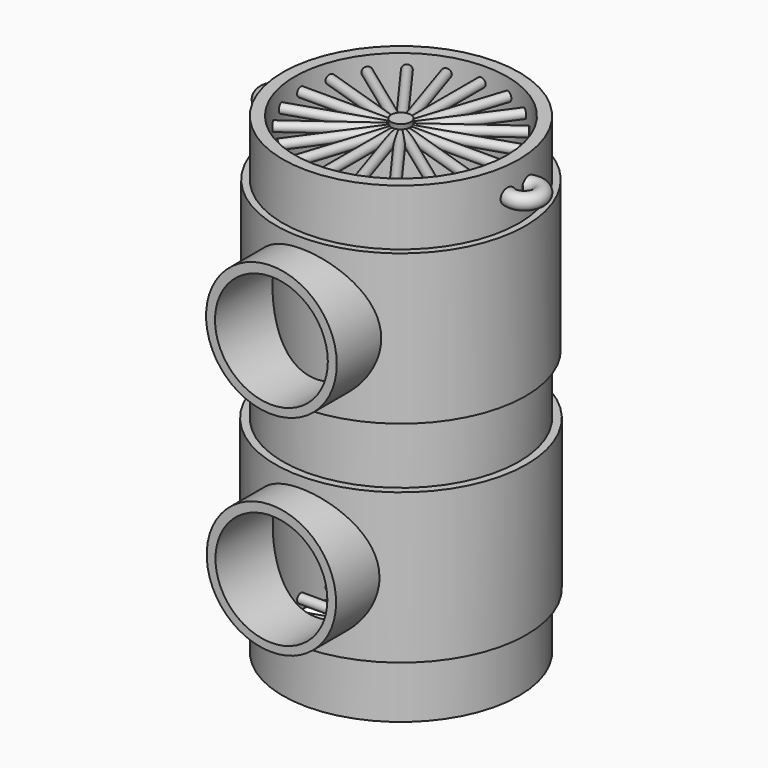
from build123d import *

# Parameters (mm, degrees)
F0_R      = 50
F1_DEPTH  = 100
F3_R      = 52.8567607849
F4_DEPTH  = 63.5
F6_R      = 53.2150165933
F7_DEPTH  = 63.5
F9_R      = 27.6777102691
F9_R_2    = 27.4003566056
F11_R     = 44.9963052647
F12_DEPTH = 104.14
F13_R     = 23.8902101051
F13_R_2   = 23.6973666463
F14_DEPTH = 30.4506270542
F16_R     = 4.1676041999
F17_DEPTH = 10
F18_R     = 1.9662297222
F19_DEPTH = 42.418
F20_COUNT = 20
F22_R     = 4.1676041999
F23_DEPTH = 10
F24_R     = 1.9662297222
F25_DEPTH = 42.418
F26_COUNT = 20
F27_R     = 3.2683339777
F31_R     = 3.2683339777


with BuildPart() as f1:
    # F0 (on Top) → F1 (new body, symmetric)
    with BuildSketch(Plane.XY):
        Circle(F0_R)
    extrude(amount=F1_DEPTH, both=True)

    # F3 (on offset) → F4 (join)
    with BuildSketch(Plane.XY.offset(12.7)):
        Circle(F3_R)
    extrude(amount=F4_DEPTH)

    # F6 (on offset) → F7 (join)
    with BuildSketch(Plane.XY.offset(-12.7)):
        Circle(F6_R)
    extrude(amount=-F7_DEPTH)

    # F9 (on offset) → F10 (join, up to the next surface of F1)
    with BuildSketch(Plane.XZ.offset(68.58)):
        with Locations((0, 44.2950055003)):
            Circle(F9_R)
        with Locations((0, -44.6592606604)):
            Circle(F9_R_2)
    extrude(until=Until.NEXT, dir=(0, 1, 0))

    # F11 (on Top) → F12 (cut, symmetric)
    with BuildSketch(Plane.XY):
        Circle(F11_R)
    extrude(amount=F12_DEPTH, both=True, mode=Mode.SUBTRACT)

    # F13 (on offset) → F14 (cut, through all)
    with BuildSketch(Plane.XZ.offset(68.58)):
        with Locations((0, 44.0187491477)):
            Circle(F13_R)
        with Locations((0, -44.9355132878)):
            Circle(F13_R_2)
    extrude(amount=-F14_DEPTH, mode=Mode.SUBTRACT)

    # F30: sweep along a path in F29
    with BuildLine(Plane.XY.offset(88.9)) as f30_path:
        ThreePointArc((47.9346827759, -4.0421244387), (58.1737168737, 0.1056825748), (47.7930903435, 3.8851951249))
    # F27 (on Front) → F30 (sweep)
    with BuildSketch(Plane.XZ):
        with Locations((58.2703016698, 88.4469673038)):
            Circle(F27_R)
    sweep(path=f30_path.line)

    # F33: sweep along a path in F32
    with BuildLine(Plane.XY.offset(88.9)) as f33_path:
        ThreePointArc((-48.183990846, 4.5897704173), (-57.4757854405, -0.0363228438), (-48.126578331, -4.5452597551))
    # F31 (on Front) → F33 (sweep)
    with BuildSketch(Plane.XZ):
        with Locations((-57.4374236166, 89.2748013139)):
            Circle(F31_R)
    sweep(path=f33_path.line)


with BuildPart() as f17:
    # F16 (on offset) → F17 (new body)
    with BuildSketch(Plane.XY.offset(99.06)):
        Circle(F16_R)
    extrude(amount=-F17_DEPTH)

    # F18 (on Front) → F19 (join)
    with BuildSketch(Plane.XZ):
        with Locations((0, 95.1355397701)):
            Circle(F18_R)
    extrude(amount=F19_DEPTH)


with BuildPart() as f20_1:
    # F20: instance of F17
    add(f17.part.rotate(Axis((0, 0, 99.06), (0, 0, 1)), 1 * 360 / F20_COUNT))


with BuildPart() as f20_2:
    # F20: instance of F17
    add(f17.part.rotate(Axis((0, 0, 99.06), (0, 0, 1)), 2 * 360 / F20_COUNT))


with BuildPart() as f20_3:
    # F20: instance of F17
    add(f17.part.rotate(Axis((0, 0, 99.06), (0, 0, 1)), 3 * 360 / F20_COUNT))


with BuildPart() as f20_4:
    # F20: instance of F17
    add(f17.part.rotate(Axis((0, 0, 99.06), (0, 0, 1)), 4 * 360 / F20_COUNT))


with BuildPart() as f20_5:
    # F20: instance of F17
    add(f17.part.rotate(Axis((0, 0, 99.06), (0, 0, 1)), 5 * 360 / F20_COUNT))


with BuildPart() as f20_6:
    # F20: instance of F17
    add(f17.part.rotate(Axis((0, 0, 99.06), (0, 0, 1)), 6 * 360 / F20_COUNT))


with BuildPart() as f20_7:
    # F20: instance of F17
    add(f17.part.rotate(Axis((0, 0, 99.06), (0, 0, 1)), 7 * 360 / F20_COUNT))


with BuildPart() as f20_8:
    # F20: instance of F17
    add(f17.part.rotate(Axis((0, 0, 99.06), (0, 0, 1)), 8 * 360 / F20_COUNT))


with BuildPart() as f20_9:
    # F20: instance of F17
    add(f17.part.rotate(Axis((0, 0, 99.06), (0, 0, 1)), 9 * 360 / F20_COUNT))


with BuildPart() as f20_10:
    # F20: instance of F17
    add(f17.part.rotate(Axis((0, 0, 99.06), (0, 0, 1)), 10 * 360 / F20_COUNT))


with BuildPart() as f20_11:
    # F20: instance of F17
    add(f17.part.rotate(Axis((0, 0, 99.06), (0, 0, 1)), 11 * 360 / F20_COUNT))


with BuildPart() as f20_12:
    # F20: instance of F17
    add(f17.part.rotate(Axis((0, 0, 99.06), (0, 0, 1)), 12 * 360 / F20_COUNT))


with BuildPart() as f20_13:
    # F20: instance of F17
    add(f17.part.rotate(Axis((0, 0, 99.06), (0, 0, 1)), 13 * 360 / F20_COUNT))


with BuildPart() as f20_14:
    # F20: instance of F17
    add(f17.part.rotate(Axis((0, 0, 99.06), (0, 0, 1)), 14 * 360 / F20_COUNT))


with BuildPart() as f20_15:
    # F20: instance of F17
    add(f17.part.rotate(Axis((0, 0, 99.06), (0, 0, 1)), 15 * 360 / F20_COUNT))


with BuildPart() as f20_16:
    # F20: instance of F17
    add(f17.part.rotate(Axis((0, 0, 99.06), (0, 0, 1)), 16 * 360 / F20_COUNT))


with BuildPart() as f20_17:
    # F20: instance of F17
    add(f17.part.rotate(Axis((0, 0, 99.06), (0, 0, 1)), 17 * 360 / F20_COUNT))


with BuildPart() as f20_18:
    # F20: instance of F17
    add(f17.part.rotate(Axis((0, 0, 99.06), (0, 0, 1)), 18 * 360 / F20_COUNT))


with BuildPart() as f20_19:
    # F20: instance of F17
    add(f17.part.rotate(Axis((0, 0, 99.06), (0, 0, 1)), 19 * 360 / F20_COUNT))


with BuildPart() as f23:
    # F22 (on offset) → F23 (new body)
    with BuildSketch(Plane.XY.offset(-98.806)):
        Circle(F22_R)
    extrude(amount=F23_DEPTH)

    # F24 (on Front) → F25 (join)
    with BuildSketch(Plane.XZ):
        with Locations((0, -93.6467796564)):
            Circle(F24_R)
    extrude(amount=F25_DEPTH)


with BuildPart() as f26_1:
    # F26: instance of F23
    add(f23.part.rotate(Axis((0, 0, -98.806), (0, 0, -1)), 1 * 360 / F26_COUNT))


with BuildPart() as f26_2:
    # F26: instance of F23
    add(f23.part.rotate(Axis((0, 0, -98.806), (0, 0, -1)), 2 * 360 / F26_COUNT))


with BuildPart() as f26_3:
    # F26: instance of F23
    add(f23.part.rotate(Axis((0, 0, -98.806), (0, 0, -1)), 3 * 360 / F26_COUNT))


with BuildPart() as f26_4:
    # F26: instance of F23
    add(f23.part.rotate(Axis((0, 0, -98.806), (0, 0, -1)), 4 * 360 / F26_COUNT))


with BuildPart() as f26_5:
    # F26: instance of F23
    add(f23.part.rotate(Axis((0, 0, -98.806), (0, 0, -1)), 5 * 360 / F26_COUNT))


with BuildPart() as f26_6:
    # F26: instance of F23
    add(f23.part.rotate(Axis((0, 0, -98.806), (0, 0, -1)), 6 * 360 / F26_COUNT))


with BuildPart() as f26_7:
    # F26: instance of F23
    add(f23.part.rotate(Axis((0, 0, -98.806), (0, 0, -1)), 7 * 360 / F26_COUNT))


with BuildPart() as f26_8:
    # F26: instance of F23
    add(f23.part.rotate(Axis((0, 0, -98.806), (0, 0, -1)), 8 * 360 / F26_COUNT))


with BuildPart() as f26_9:
    # F26: instance of F23
    add(f23.part.rotate(Axis((0, 0, -98.806), (0, 0, -1)), 9 * 360 / F26_COUNT))


with BuildPart() as f26_10:
    # F26: instance of F23
    add(f23.part.rotate(Axis((0, 0, -98.806), (0, 0, -1)), 10 * 360 / F26_COUNT))


with BuildPart() as f26_11:
    # F26: instance of F23
    add(f23.part.rotate(Axis((0, 0, -98.806), (0, 0, -1)), 11 * 360 / F26_COUNT))


with BuildPart() as f26_12:
    # F26: instance of F23
    add(f23.part.rotate(Axis((0, 0, -98.806), (0, 0, -1)), 12 * 360 / F26_COUNT))


with BuildPart() as f26_13:
    # F26: instance of F23
    add(f23.part.rotate(Axis((0, 0, -98.806), (0, 0, -1)), 13 * 360 / F26_COUNT))


with BuildPart() as f26_14:
    # F26: instance of F23
    add(f23.part.rotate(Axis((0, 0, -98.806), (0, 0, -1)), 14 * 360 / F26_COUNT))


with BuildPart() as f26_15:
    # F26: instance of F23
    add(f23.part.rotate(Axis((0, 0, -98.806), (0, 0, -1)), 15 * 360 / F26_COUNT))


with BuildPart() as f26_16:
    # F26: instance of F23
    add(f23.part.rotate(Axis((0, 0, -98.806), (0, 0, -1)), 16 * 360 / F26_COUNT))


with BuildPart() as f26_17:
    # F26: instance of F23
    add(f23.part.rotate(Axis((0, 0, -98.806), (0, 0, -1)), 17 * 360 / F26_COUNT))


with BuildPart() as f26_18:
    # F26: instance of F23
    add(f23.part.rotate(Axis((0, 0, -98.806), (0, 0, -1)), 18 * 360 / F26_COUNT))


with BuildPart() as f26_19:
    # F26: instance of F23
    add(f23.part.rotate(Axis((0, 0, -98.806), (0, 0, -1)), 19 * 360 / F26_COUNT))


solid = Compound([f1.part, f17.part, f20_1.part, f20_2.part, f20_3.part, f20_4.part, f20_5.part, f20_6.part, f20_7.part, f20_8.part, f20_9.part, f20_10.part, f20_11.part, f20_12.part, f20_13.part, f20_14.part, f20_15.part, f20_16.part, f20_17.part, f20_18.part, f20_19.part, f23.part, f26_1.part, f26_2.part, f26_3.part, f26_4.part, f26_5.part, f26_6.part, f26_7.part, f26_8.part, f26_9.part, f26_10.part, f26_11.part, f26_12.part, f26_13.part, f26_14.part, f26_15.part, f26_16.part, f26_17.part, f26_18.part, f26_19.part])
